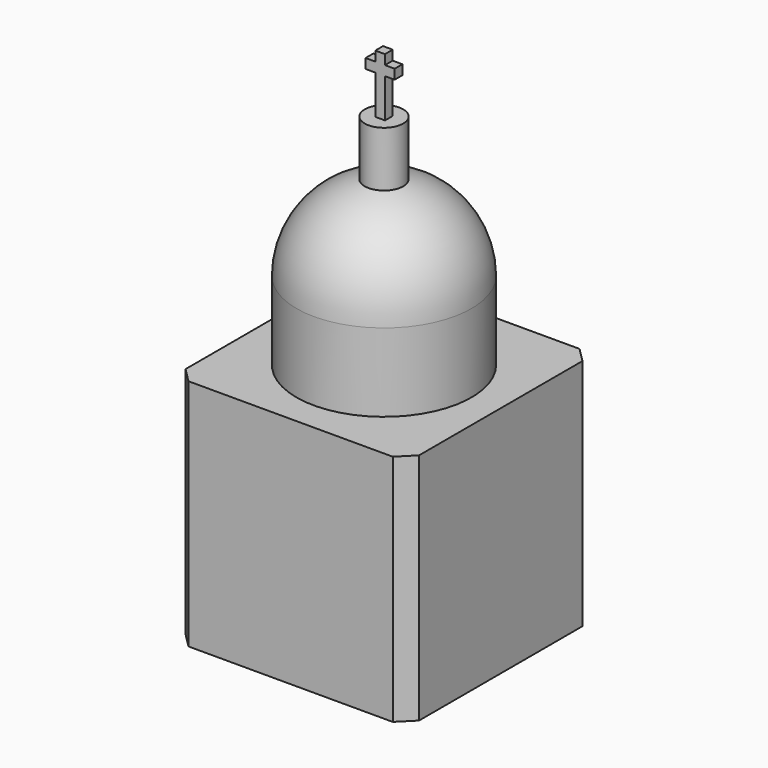
from build123d import *

# Parameters (mm, degrees)
F0_W     = 50.8
F0_H     = 50.8
F1_DEPTH = 50.8
F2_SIZE  = 3.175
F3_W     = 19.05
F3_H     = 17.018
F5_W     = 2.1082
F5_H     = 2.1082
F6_DEPTH = 1.0541


with BuildPart() as f1:
    # F0 (on Top) → F1 (new body)
    with BuildSketch(Plane.XY):
        Rectangle(F0_W, F0_H)
    extrude(amount=F1_DEPTH)

    # F2
    f2_edges = [f1.edges().sort_by_distance(p)[0] for p in [
        (25.4, -25.4, 25.4),
        (25.4, 25.4, 25.4),
        (-25.4, 25.4, 25.4),
        (-25.4, -25.4, 25.4),
    ]]
    chamfer(f2_edges, length=F2_SIZE)

    # F3 (on Front) → F4 (revolve)
    with BuildSketch(Plane.XZ):
        with Locations((-9.525, 59.309)):
            Rectangle(F3_W, F3_H)
        with BuildLine():
            Line((-19.05, 67.818), (0, 67.818))
            Line((0, 67.818), (0, 86.4012725589))
            Line((0, 86.4012725589), (-4.191, 86.4012725589))
            ThreePointArc((-4.191, 86.4012725589), (-14.8785256326, 79.7147211869), (-19.05, 67.818))
        make_face()
        Polygon((-4.191, 86.4012725589), (0, 86.4012725589), (0, 86.868), (0, 98.425), (-4.191, 98.425), align=None)
    revolve(axis=Axis((0, 0, 59.309), (0, 0, 1)))

    # F5 (on Front) → F6 (join, symmetric)
    with BuildSketch(Plane.XZ):
        with Locations((-2.1082, 107.9627)):
            Rectangle(F5_W, F5_H)
        Polygon((-1.0541, 98.425), (0, 98.425), (0, 111.125), (-1.0541, 111.125), (-1.0541, 109.0168), (-1.0541, 106.9086), align=None)
    extrude(amount=F6_DEPTH, both=True)

    # F7: F1 across face


with BuildPart() as f1_1:
    add(f1.part)
    add(f1.part.mirror(Plane(origin=(0, 0, 104.775), x_dir=(0, 1, 0), z_dir=(1, 0, 0))))


solid = f1_1.part
